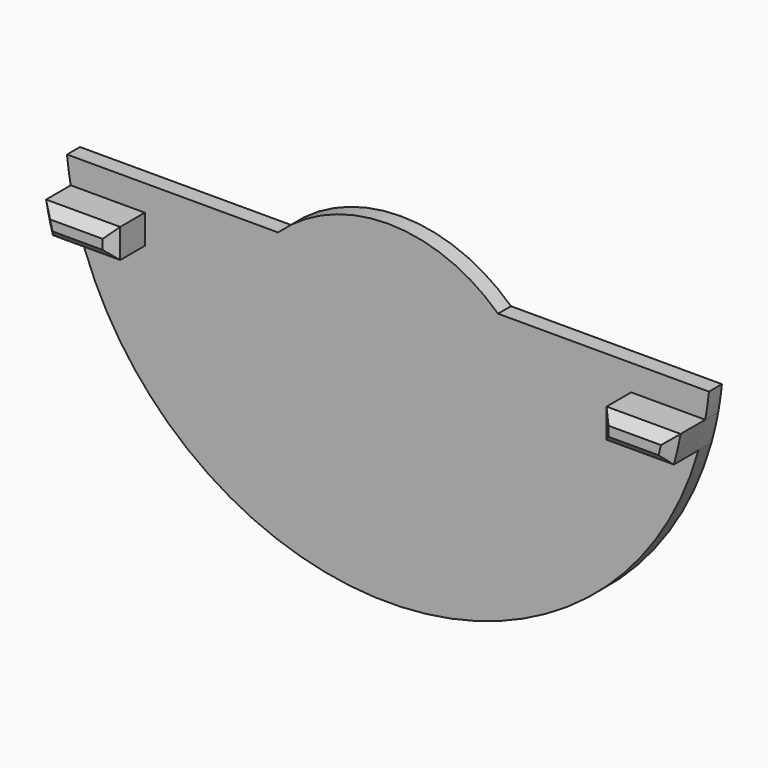
from build123d import *

# Parameters (mm, degrees)
F1_DEPTH = 1.27
F2_DEPTH = 4.445
F3_SIZE2 = 0.762
F3_SIZE  = 0.762


# Not quite as in the source:
# - a feature names something its author has since deleted; it is built from what else it names


with BuildPart() as f1:
    # F0 (on Front) → F1 (new body)
    with BuildSketch(Plane.XZ):
        with BuildLine():
            Line((-8.6160342025, -3.05308), (-25.146, -3.05308))
            ThreePointArc((-25.146, -3.05308), (-25.0213724382, -4.0720308287), (-24.855468258, -5.08508))
            Line((-24.855468258, -5.08508), (-19.05, -5.08508))
            Line((-19.05, -5.08508), (-19.05, -7.37108))
            Line((-19.05, -7.37108), (-24.3224034139, -7.37108))
            ThreePointArc((-24.3224034139, -7.37108), (-0.002803144, -25.7679203368), (24.3167971258, -7.37108))
            Line((24.3167971258, -7.37108), (19.05, -7.37108))
            Line((19.05, -7.37108), (19.05, -5.08508))
            Line((19.05, -5.08508), (24.8498619699, -5.08508))
            ThreePointArc((24.8498619699, -5.08508), (25.0157661502, -4.0720308287), (25.1403937119, -3.05308))
            Line((25.1403937119, -3.05308), (8.6160342025, -3.05308))
            ThreePointArc((8.6160342025, -3.05308), (11.5583898274, -7.2348059893), (12.5961765249, -12.2415302321))
            ThreePointArc((12.5961765249, -12.2415302321), (-5.0067242428, -23.7999200595), (-8.6160342025, -3.05308))
        make_face()
        with BuildLine():
            Line((8.6160342025, -3.05308), (-8.6160342025, -3.05308))
            ThreePointArc((-8.6160342025, -3.05308), (-5.0067242428, -23.7999200595), (12.5961765249, -12.2415302321))
            ThreePointArc((12.5961765249, -12.2415302321), (11.5583898274, -7.2348059893), (8.6160342025, -3.05308))
        make_face()
        with BuildLine():
            ThreePointArc((8.6160342025, -3.05308), (0, 0.3546462928), (-8.6160342025, -3.05308))
            Line((-8.6160342025, -3.05308), (8.6160342025, -3.05308))
        make_face()
    extrude(amount=F1_DEPTH)

    # F0 (on Front) → F2 (join)
    with BuildSketch(Plane.XZ):
        with BuildLine():
            Line((-19.05, -5.08508), (-24.855468258, -5.08508))
            ThreePointArc((-24.855468258, -5.08508), (-24.6154903144, -6.2342721517), (-24.3224034139, -7.37108))
            Line((-24.3224034139, -7.37108), (-19.05, -7.37108))
            Line((-19.05, -7.37108), (-19.05, -5.08508))
        make_face()
        with BuildLine():
            Line((19.05, -7.37108), (24.3167971258, -7.37108))
            ThreePointArc((24.3167971258, -7.37108), (24.6098840263, -6.2342721517), (24.8498619699, -5.08508))
            Line((24.8498619699, -5.08508), (19.05, -5.08508))
            Line((19.05, -5.08508), (19.05, -7.37108))
        make_face()
    extrude(amount=F2_DEPTH)

    # F3
    f3_edges = [f1.edges().sort_by_distance(p)[0] for p in [
        (21.949931, -4.445, -5.08508),
        (19.05, -4.445, -6.22808),
        (21.683399, -4.445, -7.37108),
        (24.609884, -4.445, -6.234272),
        (-21.686202, -4.445, -7.37108),
        (-24.61549, -4.445, -6.234272),
        (-19.05, -4.445, -6.22808),
        (-21.952734, -4.445, -5.08508),
    ]]
    chamfer(f3_edges, length=F3_SIZE, length2=F3_SIZE2)


solid = f1.part
